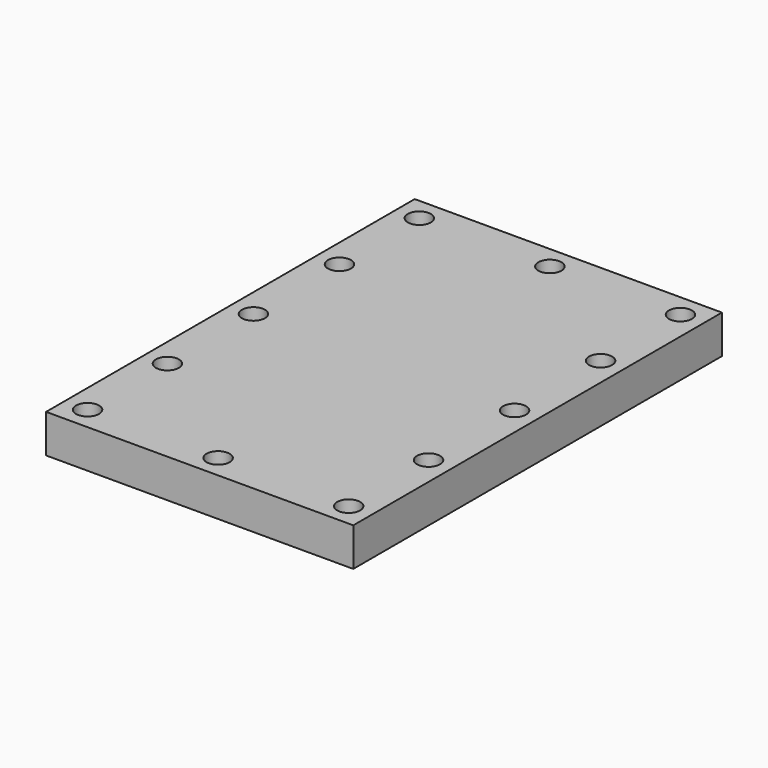
from build123d import *

# Parameters (mm, degrees)
F0_W     = 100
F0_H     = 150
F1_DEPTH = 12.5
F2_R     = 3.75
F3_DEPTH = 25


# Not quite as in the source:
# - a feature names something its author has since deleted; it is built from what else it names


with BuildPart() as f1:
    # F0 (on Top) → F1 (new body)
    with BuildSketch(Plane.XY):
        Rectangle(F0_W, F0_H)
    extrude(amount=F1_DEPTH)

    # F2 (on face) → F3 (cut)
    with BuildSketch(Plane.XY.offset(12.5)):
        with Locations((-42.5, 67.5)):
            Circle(F2_R)
        with Locations((-42.5, 0)):
            Circle(F2_R)
        with Locations((-42.5, -35)):
            Circle(F2_R)
        with Locations((-42.5, -67.5)):
            Circle(F2_R)
        with Locations((0, -67.5)):
            Circle(F2_R)
        with Locations((-42.5, 35)):
            Circle(F2_R)
        with Locations((42.5, -67.5)):
            Circle(F2_R)
        with Locations((42.5, -35)):
            Circle(F2_R)
        with Locations((42.5, 0)):
            Circle(F2_R)
        with Locations((42.5, 35)):
            Circle(F2_R)
        with Locations((42.5, 67.5)):
            Circle(F2_R)
        with Locations((0, 67.5)):
            Circle(F2_R)
    extrude(amount=-F3_DEPTH, mode=Mode.SUBTRACT)


solid = f1.part
